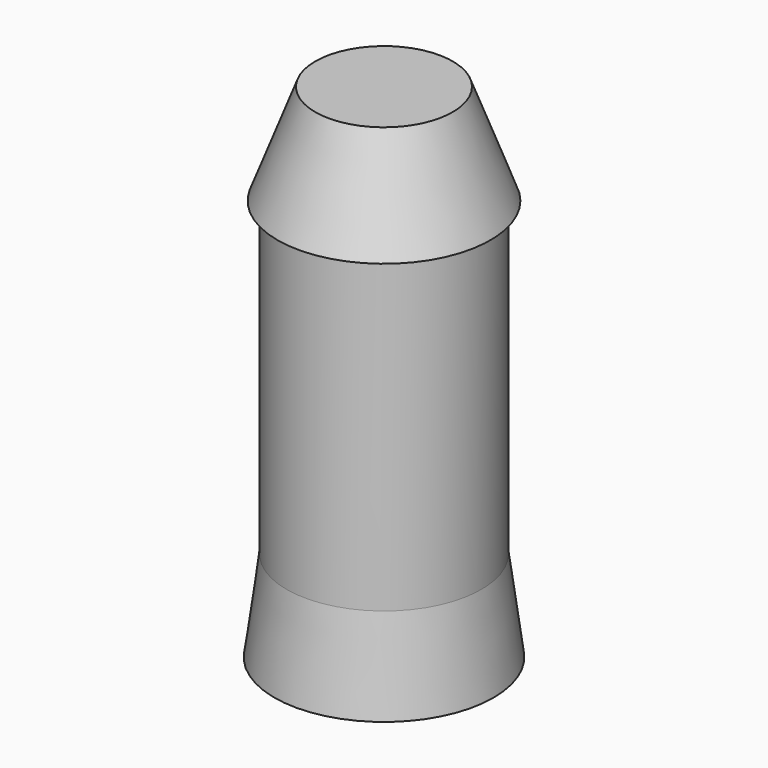
from build123d import *

# Parameters (mm, degrees)
F0_W = 3.2
F0_H = 5.1


# Not quite as in the source:
# - a feature names something its author has since deleted; it is built from what else it names


with BuildPart() as f1:
    # F0 (on Front) → F1 (revolve)
    with BuildSketch(Plane.XZ):
        Polygon((-3.2, 5.1), (0, 5.1), (0, 8.4), (-2.2580645161, 8.4), (-3.5, 5.1), align=None)
        with Locations((-1.6, 2.55)):
            Rectangle(F0_W, F0_H)
        with Locations((-1.6, -2.55)):
            Rectangle(F0_W, F0_H)
        Polygon((0, -8.1), (0, -5.1), (-3.2, -5.1), (-3.6, -8.1), align=None)
    revolve(axis=Axis((0, 0, -2.55), (0, 0, -1)))


solid = f1.part
